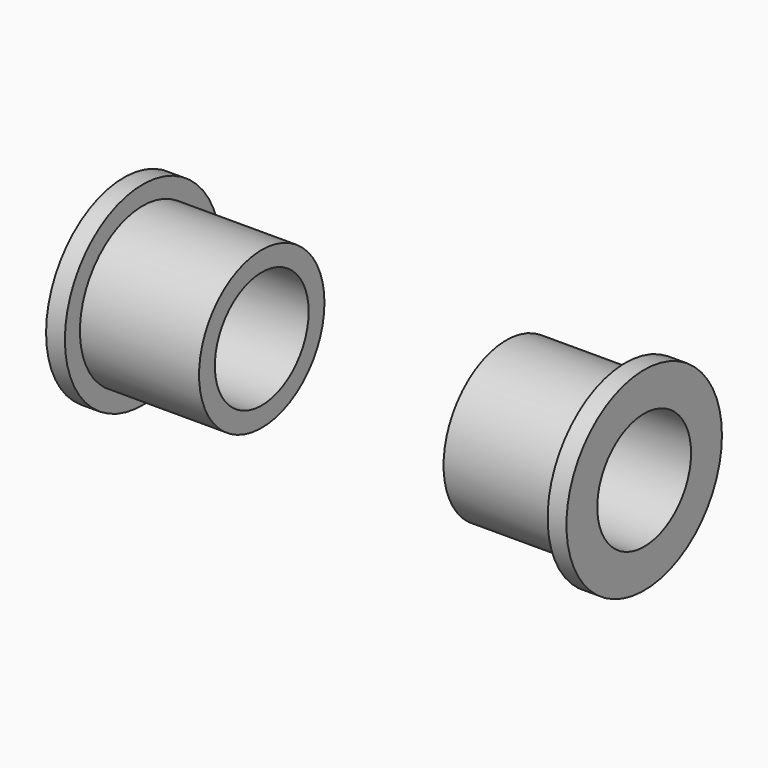
from build123d import *

# Parameters (mm, degrees)
F0_R     = 3.175
F0_R_2   = 2.3749
F1_DEPTH = 9.779
F2_R     = 3.937
F2_R_2   = 3.175
F2_R_3   = 2.3749
F3_DEPTH = 0.762
F4_R     = 3.937
F4_R_2   = 3.175
F4_R_3   = 2.3749
F5_DEPTH = 0.762
F6_W     = 9.906
F6_H     = 12.6722976956
F7_DEPTH = 12.7


with BuildPart() as f1:
    # F0 (on Right) → F1 (new body, symmetric)
    with BuildSketch(Plane.YZ):
        Circle(F0_R)
        Circle(F0_R_2, mode=Mode.SUBTRACT)
    extrude(amount=F1_DEPTH, both=True)

    # F2 (on face) → F3 (join)
    with BuildSketch(Plane.YZ.offset(9.779)):
        Circle(F2_R)
        Circle(F2_R_2, mode=Mode.SUBTRACT)
        Circle(F2_R_2)
        Circle(F2_R_3, mode=Mode.SUBTRACT)
    extrude(amount=F3_DEPTH)

    # F4 (on face) → F5 (join)
    with BuildSketch(Plane(origin=(-9.779, 0, 0), x_dir=(0, -1, 0), z_dir=(-1, 0, 0))):
        Circle(F4_R)
        Circle(F4_R_2, mode=Mode.SUBTRACT)
        Circle(F4_R_2)
        Circle(F4_R_3, mode=Mode.SUBTRACT)
    extrude(amount=F5_DEPTH)

    # F6 (on Front) → F7 (cut, symmetric)
    with BuildSketch(Plane.XZ):
        Rectangle(F6_W, F6_H)
    extrude(amount=F7_DEPTH, both=True, mode=Mode.SUBTRACT)


solid = f1.part
